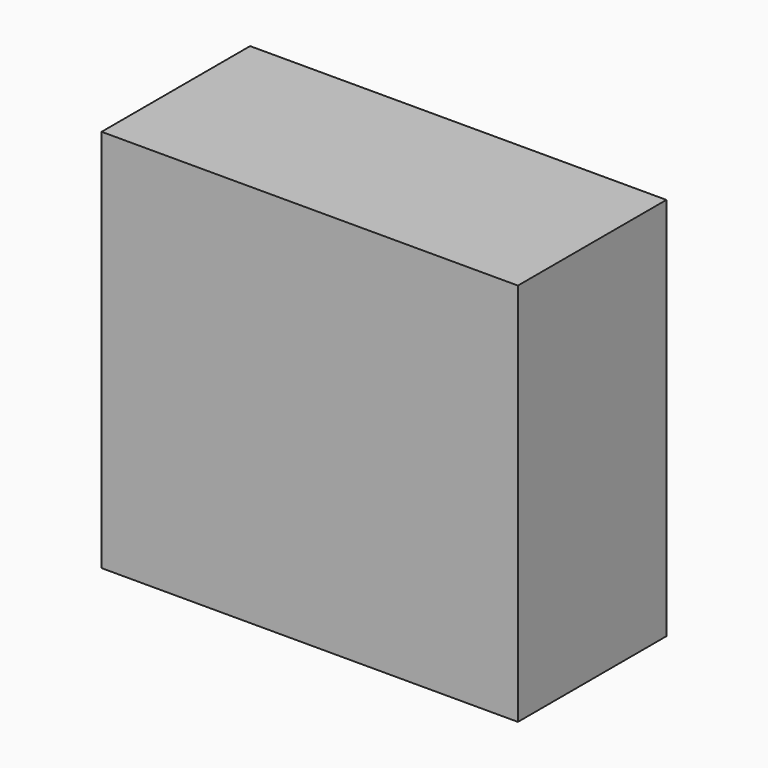
from build123d import *

# Parameters (mm, degrees)
F0_W     = 56.0792163014
F0_H     = 51.7431944609
F1_DEPTH = 25


# Not quite as in the source:
# - the program builds the solid bodies; features that only make, move or delete a surface that nothing else refers to are left out


with BuildPart() as f1:
    # F0 (on Front) → F1 (new body)
    with BuildSketch(Plane.XZ):
        with Locations((-38.5905914009, 0)):
            Rectangle(F0_W, F0_H)
    extrude(amount=F1_DEPTH)


solid = f1.part
